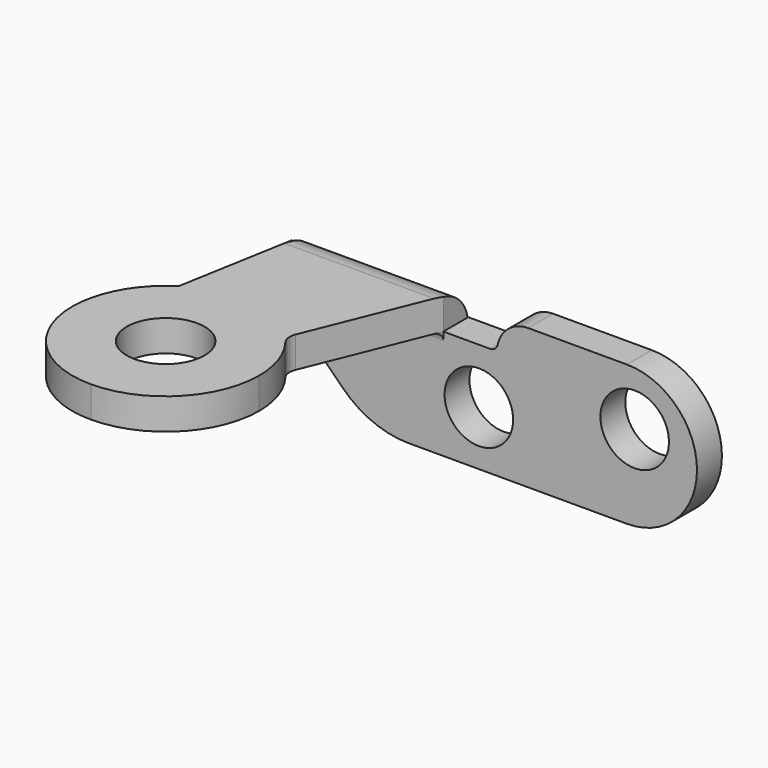
from build123d import *

# Parameters (mm, degrees)
F1_DEPTH     = 2
F2_D         = 4.4
F3_W         = 13.8216872486
F3_H         = 2
F4_DEPTH     = 20.5
F5_R         = 2.5
F6_DEPTH     = 25
F7_R         = 1
F8_T4_DEPTH  = 12.2216872486
F8_T10_DEPTH = 12.2216872486
F8_S11_R     = 2
F8_T12_DEPTH = 8
F10_DEPTH    = 9.7216872486


# Not quite as in the source:
# - a fillet or chamfer that OpenCascade refuses, or shapes differently, is made with other operations: its cross-section is extruded or revolved along the edge and cut away or added


with BuildPart() as f1:
    # F0 (on Front) → F1 (new body)
    with BuildSketch(Plane.XZ):
        with BuildLine():
            Line((-5.5351668461, -4.5), (8.4648331539, -4.5))
            ThreePointArc((8.4648331539, -4.5), (12.9648331539, 0), (8.4648331539, 4.5))
            Line((8.4648331539, 4.5), (2.1292536968, 4.5))
            ThreePointArc((2.1292536968, 4.5), (0.8745117295, 4.0574410408), (0.1750670613, 2.9256225954))
            ThreePointArc((0.1750670613, 2.9256225954), (0.0002058943, 2.6426679841), (-0.3134795975, 2.5320282443))
            Line((-0.3134795975, 2.5320282443), (-13.0351668461, 2.5320282443))
            ThreePointArc((-13.0351668461, 2.5320282443), (-13.2536814771, 1.2929397336), (-12.6890072408, 0.1685590205))
            Line((-12.6890072408, 0.1685590205), (-9.7778075332, -2.7426406871))
            ThreePointArc((-9.7778075332, -2.7426406871), (-7.8312674403, -4.0432771951), (-5.5351668461, -4.5))
        make_face()
    extrude(amount=F1_DEPTH)

    # F2 (through all)
    with Locations(Plane(origin=(0, 0, 0), x_dir=(1, 0, 0), z_dir=(0, 1, 0))):
        with Locations((-1.0351668461, 1), (8.9648331539, -1)):
            Hole(F2_D / 2)

    # F3 (on face) → F4 (join)
    with BuildSketch(Plane(origin=(0, 0, 0), x_dir=(-1, 0, 0), z_dir=(0, 1, 0))):
        with Locations((10.2243232218, 3.5320282443)):
            Rectangle(F3_W, F3_H)
    extrude(amount=-F4_DEPTH)

    # F5 (on face) → F6 (cut)
    with BuildSketch(Plane(origin=(0, 0, 2.5320282443), x_dir=(1, 0, 0), z_dir=(0, 0, -1))):
        with BuildLine():
            Line((-6.7216205274, 10.43544481), (-3.3134795975, 2))
            Line((-3.3134795975, 2), (-3.3134795975, 20.5))
            Line((-3.3134795975, 20.5), (-11.1351668461, 20.5))
            ThreePointArc((-11.1351668461, 20.5), (-6.892526159, 18.7426406871), (-5.1351668461, 14.5))
            ThreePointArc((-5.1351668461, 14.5), (-5.5458342423, 12.3184040145), (-6.7216205274, 10.43544481))
        make_face()
        with BuildLine():
            Line((-17.1351668461, 20.5), (-17.1351668461, 14.5))
            ThreePointArc((-17.1351668461, 14.5), (-15.3778075332, 18.7426406871), (-11.1351668461, 20.5))
            Line((-11.1351668461, 20.5), (-17.1351668461, 20.5))
        make_face()
        with BuildLine():
            Line((-17.1351668461, 0), (-13.0351668461, 0))
            Line((-13.0351668461, 0), (-13.0351668461, 2))
            Line((-13.0351668461, 2), (-14.3454662645, 9.4310772699))
            ThreePointArc((-14.3454662645, 9.4310772699), (-16.3916769293, 11.6070600171), (-17.1351668461, 14.5))
            Line((-17.1351668461, 14.5), (-17.1351668461, 0))
        make_face()
        with Locations((-11.1351668461, 14.5)):
            Circle(F5_R)
    extrude(amount=-F6_DEPTH, mode=Mode.SUBTRACT)

    # F7
    f7_edges = [f1.edges().sort_by_distance(p)[0] for p in [
        (-6.721621, -10.435445, 3.532028),
    ]]
    fillet(f7_edges, radius=F7_R)

    # F8: fillet of radius 0.5 on 1 edges, made by hand


with BuildPart() as f8_tool2:
    # F8_s3 → F8_t4 (new body)
    with BuildSketch(Plane.YZ.offset(-2.0634795975)):
        with BuildLine():
            ThreePointArc((-2.5, 2.5320282443), (-2.1464466094, 2.3855816349), (-2, 2.0320282443))
            Line((-2, 2.0320282443), (-2, 2.5320282443))
            Line((-2, 2.5320282443), (-2.5, 2.5320282443))
        make_face()
    extrude(amount=-F8_T4_DEPTH)

    split(bisect_by=Plane(origin=(-2.1538403044, 0.8702079692, 0), x_dir=(0, 0, 1), z_dir=(-0.9271838546, 0.3746065934, 0)), keep=Keep.TOP)

    split(bisect_by=Plane(origin=(-12.3000883277, 2.1688374373, 0), x_dir=(0, 0, 1), z_dir=(0.984807753, -0.1736481777, 0)), keep=Keep.TOP)


with BuildPart() as f1_1:
    add(f1.part)

    # F8_t1: union F8_tool2
    add(f8_tool2.part)


with BuildPart() as f8_tool8:
    # F8_s9 → F8_t10 (new body)
    with BuildSketch(Plane.YZ.offset(-2.0634795975)):
        with BuildLine():
            ThreePointArc((-2.5, 2.5320282443), (-2.1464466094, 2.3855816349), (-2, 2.0320282443))
            Line((-2, 2.0320282443), (-2, 2.5320282443))
            Line((-2, 2.5320282443), (-2.5, 2.5320282443))
        make_face()
    extrude(amount=-F8_T10_DEPTH)

    # F8_s11 → F8_t12 (intersect, symmetric)
    with BuildSketch(Plane.XZ.offset(2.2)):
        with Locations((-11.2747936785, 1.5827725829)):
            Circle(F8_S11_R)
    extrude(amount=F8_T12_DEPTH, both=True, mode=Mode.INTERSECT)


with BuildPart() as f1_2:
    add(f1_1.part)

    # F8_t7: union F8_tool8
    add(f8_tool8.part)

    # F9 (on face) → F10 (cut, through all)
    with BuildSketch(Plane(origin=(-13.0351668461, 0, 0), x_dir=(0, -1, 0), z_dir=(-1, 0, 0))):
        with BuildLine():
            Line((2.5, 4.5320282443), (2, 4.5320282443))
            Line((2, 4.5320282443), (0, 4.5320282443))
            Line((0, 4.5320282443), (0, 2.5320282443))
            Line((0, 2.5320282443), (0, 2.0320282443))
            ThreePointArc((0, 2.0320282443), (0.732233047, 3.7997951973), (2.5, 4.5320282443))
        make_face()
    extrude(amount=-F10_DEPTH, mode=Mode.SUBTRACT)


solid = f1_2.part
